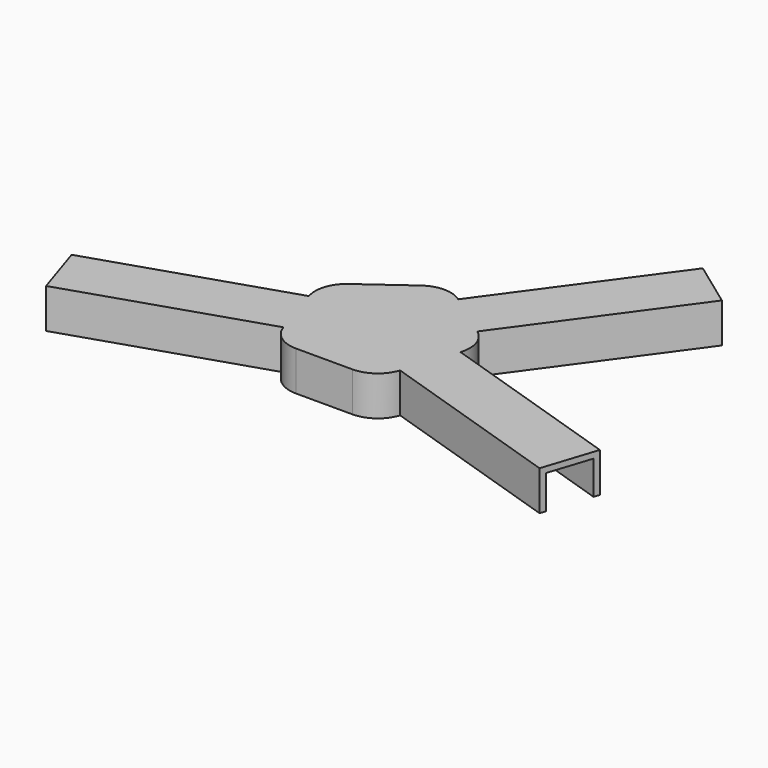
from build123d import *

# Parameters (mm, degrees)
F1_DEPTH      = 10
F2_R          = 8
F3_T          = -1.5
F4_W          = 14.2378706528
F4_H          = 10
F5_DEPTH      = 50
F7_W          = 14.2378706528
F7_H          = 10
F8_DEPTH      = 50
F6_W          = 14.2378706528
F6_H          = 10
F9_DEPTH      = 50
F10_T         = 1.5
F10_T3_DEPTH  = 13
F10_T5_DEPTH  = 17.2378706528
F10_T7_DEPTH  = 17.2378706528
F10_T10_ANGLE = 72.000000001
F10_T12_ANGLE = 72.000000001
F10_T14_ANGLE = 72.000000001
F10_T16_ANGLE = 72.000000001
F10_T18_ANGLE = 72.000000001


# Not quite as in the source:
# - a shell that OpenCascade refuses in one call is made with other operations: the cavity is built on its own and cut out


with BuildPart() as f1:
    # F0 (on Top) → F1 (new body)
    with BuildSketch(Plane.XY):
        Polygon((20.9232433585, 6.7983738762), (0, 22), (-20.9232433585, 6.7983738762), (-12.9312755504, -17.7983738762), (12.9312755504, -17.7983738762), align=None)
    extrude(amount=F1_DEPTH)

    # F2
    f2_edges = [f1.edges().sort_by_distance(p)[0] for p in [
        (20.923243, 6.798374, 5),
        (0, 22, 5),
        (12.931276, -17.798374, 5),
        (-12.931276, -17.798374, 5),
        (-20.923243, 6.798374, 5),
    ]]
    fillet(f2_edges, radius=F2_R)

    # F3
    f3_openings = [f1.faces().sort_by_distance(p)[0] for p in [
        (0, 0, 0),
    ]]
    offset(amount=F3_T, openings=f3_openings)

    # F4 (on face) → F5 (join)
    with BuildSketch(Plane(origin=(16.9272594545, -5.5, 0), x_dir=(0.3090169944, 0.9510565163, 0), z_dir=(0.9510565163, -0.3090169944, 0))):
        with Locations((0, 5)):
            Rectangle(F4_W, F4_H)
    extrude(amount=F5_DEPTH)

    # F7 (on face) → F8 (join)
    with BuildSketch(Plane(origin=(10.4616216792, 14.3991869381, 0), x_dir=(-0.8090169944, 0.5877852523, 0), z_dir=(0.5877852523, 0.8090169944, 0))):
        with Locations((0, 5)):
            Rectangle(F7_W, F7_H)
    extrude(amount=F8_DEPTH)

    # F6 (on face) → F9 (join)
    with BuildSketch(Plane(origin=(-16.9272594545, -5.5, 0), x_dir=(0.3090169944, -0.9510565163, 0), z_dir=(-0.9510565163, -0.3090169944, 0))):
        with Locations((0, 5)):
            Rectangle(F6_W, F6_H)
    extrude(amount=F9_DEPTH)

    # F10: shell of thickness 1.5, made by hand


with BuildPart() as f10_core1:
    # F10_t2: copy of F1
    add(f1.part)

    # the walls: a layer under each face that stays
    f10_faces = [f10_core1.faces().sort_by_distance(p)[0] for p in [
        (0, 20.11145618, 5),
        (-10.4616216792, 14.3991869381, 5),
        (-19.1271314522, 6.2147817412, 5),
        (-11.8212173447, -16.2705098312, 5),
        (0, -17.7983738762, 5),
        (11.8212173447, -16.2705098312, 5),
        (38.5038003641, -19.9959346906, 5),
        (42.9035443596, -6.4549150281, 5),
        (19.1271314522, 6.2147817412, 5),
        (30.9155926475, 30.4402066006, 5),
        (19.3969133257, 38.8090169944, 5),
        (17.7005466777, 5.7512562497, 4.25),
        (10.9395394663, -15.0569843397, 4.25),
        (0, -16.2983738762, 4.25),
        (-10.9395394663, -15.0569843397, 4.25),
        (-17.7005466777, 5.7512562497, 4.25),
        (-9.5799438008, 13.1856614466, 4.25),
        (0, 18.61145618, 4.25),
        (0, 15.6565411519, 10),
        (-42.9035443596, -6.4549150281, 5),
        (-38.5038003641, -19.9959346906, 5),
        (0, 1.1565411519, 8.5),
    ]]
    thicken(f10_faces, amount=-F10_T, mode=Mode.SUBTRACT)

    # F10_s4 → F10_t3 (cut)
    with BuildSketch(Plane.XY.offset(-1.5)):
        Polygon((4.6989635422, 18.6045441687), (3.8206041399, 17.3700666434), (5.0341296315, 16.488388765), (5.9158075099, 17.7019142566), align=None)
        Polygon((-19.1460325548, 1.2801404241), (-17.7005466777, 1.7340353228), (-17.2370211862, 0.3074505484), (-18.6636059606, -0.1560749432), align=None)
        Polygon((-14.7370180496, -12.2894109339), (-13.3008026823, -11.8069843397), (-13.7643281739, -10.3803995652), (-15.1909129483, -10.8439250568), align=None)
        Polygon((14.7370180496, -12.2894109339), (13.3008026823, -11.8069843397), (13.7643281739, -10.3803995652), (15.1909129483, -10.8439250568), align=None)
        Polygon((19.1460325548, 1.2801404241), (18.6636059606, -0.1560749432), (17.2370211862, 0.3074505484), (17.7005466777, 1.7340353228), align=None)
        Polygon((16.2419133739, 10.2181002174), (15.3392834617, 9.0012562497), (14.1257579702, 9.8829341281), (15.0074358486, 11.0964596197), align=None)
    extrude(amount=F10_T3_DEPTH, mode=Mode.SUBTRACT)

    # F10_s6 → F10_t5 (cut)
    with BuildSketch(Plane.YZ.offset(-8.6189353264)):
        Polygon((-16.2833738762, 8.485), (-17.7983738762, 8.5), (-17.7983738762, 10), (-16.2983738762, 10), align=None)
    extrude(amount=F10_T5_DEPTH, mode=Mode.SUBTRACT)

    # F10_s8 → F10_t7 (cut)
    with BuildSketch(Plane(origin=(6.9728651525, 5.0660830753, 0), x_dir=(0, 0, 1), z_dir=(-0.8090169944, -0.5877852523, 0))):
        Polygon((8.485, 16.2833738762), (8.5, 17.7983738762), (10, 17.7983738762), (10, 16.2983738762), align=None)
    extrude(amount=F10_T7_DEPTH, mode=Mode.SUBTRACT)

    # F10_s9 → F10_t10 (revolve, cut)
    with BuildSketch(Plane(origin=(2.1998719977, 6.7705098312, 0), x_dir=(0, 0, 1), z_dir=(-0.3090169944, -0.9510565163, 0))):
        Polygon((8.485, -16.2833738762), (8.5, -17.7983738762), (10, -17.7983738762), (10, -16.2983738762), align=None)
    revolve(axis=Axis((11.5186793218, 3.7426457862, 8.5), (0, 0, 1)), revolution_arc=F10_T10_ANGLE, mode=Mode.SUBTRACT)

    # F10_s11 → F10_t12 (revolve, cut)
    with BuildSketch(Plane.YZ.offset(7.1189353264)):
        Polygon((-16.2833738762, 8.485), (-17.7983738762, 8.5), (-17.7983738762, 10), (-16.2983738762, 10), align=None)
    revolve(axis=Axis((7.1189353264, -9.7983738762, 8.5), (0, 0, 1)), revolution_arc=F10_T12_ANGLE, mode=Mode.SUBTRACT)

    # F10_s13 → F10_t14 (revolve, cut)
    with BuildSketch(Plane(origin=(2.1998719977, -6.7705098312, 0), x_dir=(0, 0, 1), z_dir=(-0.3090169944, 0.9510565163, 0))):
        Polygon((8.485, -16.2833738762), (8.5, -17.7983738762), (10, -17.7983738762), (10, -16.2983738762), align=None)
    revolve(axis=Axis((-7.1189353264, -9.7983738762, 8.5), (0, 0, 1)), revolution_arc=F10_T14_ANGLE, mode=Mode.SUBTRACT)

    # F10_s15 → F10_t16 (revolve, cut)
    with BuildSketch(Plane(origin=(-5.7593396609, -4.1844051969, 0), x_dir=(0, 0, 1), z_dir=(0.8090169944, 0.5877852523, 0))):
        Polygon((8.485, -16.2833738762), (8.5, -17.7983738762), (10, -17.7983738762), (10, -16.2983738762), align=None)
    revolve(axis=Axis((-11.5186793218, 3.7426457862, 8.5), (0, 0, 1)), revolution_arc=F10_T16_ANGLE, mode=Mode.SUBTRACT)

    # F10_s17 → F10_t18 (revolve, cut)
    with BuildSketch(Plane(origin=(-5.7593396609, 4.1844051969, 0), x_dir=(0, 0, 1), z_dir=(0.8090169944, -0.5877852523, 0))):
        Polygon((8.485, -16.2833738762), (8.5, -17.7983738762), (10, -17.7983738762), (10, -16.2983738762), align=None)
    revolve(axis=Axis((0, 12.11145618, 8.5), (0, 0, 1)), revolution_arc=F10_T18_ANGLE, mode=Mode.SUBTRACT)


with BuildPart() as f1_1:
    add(f1.part)

    # what is left inside the walls is the cavity
    f10_cavity = [f10_core1.part.solids().sort_by_distance(p)[0] for p in [
        (24.715414, 25.972877, 0.015),
        (39.99038, -17.427366, 0.015),
        (-39.99038, -17.427366, 0.015),
    ]]
    add(f10_cavity, mode=Mode.SUBTRACT)


solid = f1_1.part
